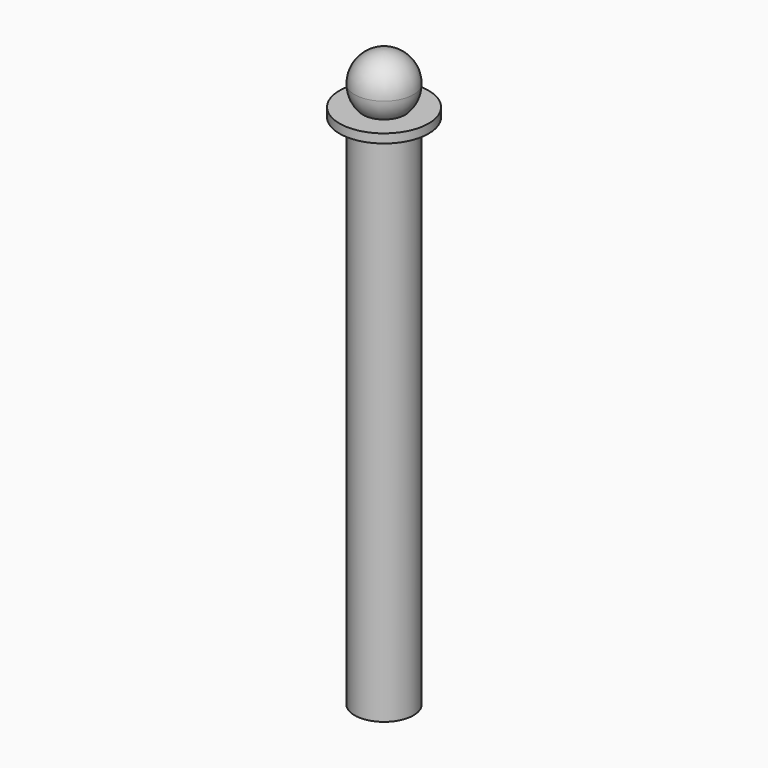
from build123d import *

# Parameters (mm, degrees)
F0_R     = 4.191
F1_DEPTH = 73.66
F2_R     = 4.191
F3_DEPTH = 8.382
F4_R     = 4.19099
F5_R     = 6.35
F6_DEPTH = 1.27
F7_R     = 1.905
F8_DEPTH = 12.7


# Not quite as in the source:
# - a fillet or chamfer is up to 0.001 mm smaller than in the source, because OpenCascade refuses the exact size


with BuildPart() as f1:
    # F0 (on Top) → F1 (new body)
    with BuildSketch(Plane.XY):
        Circle(F0_R)
    extrude(amount=F1_DEPTH)



with BuildPart() as f3:
    # F2 (on face) → F3 (new body)
    with BuildSketch(Plane.XY.offset(73.66)):
        Circle(F2_R)
    extrude(amount=F3_DEPTH)

    # F4 (radius 4.191 in the source; OpenCascade refuses exactly that, so slightly less here)
    f4_edges = [f3.edges().sort_by_distance(p)[0] for p in [
        (-4.191, 0, 73.66),
        (-4.191, 0, 82.042),
    ]]
    fillet(f4_edges, radius=F4_R)


with BuildPart() as f1_1:
    add(f1.part)

    add(f3.part)  # F6 merges F3
    # F5 (on face) → F6 (join)
    with BuildSketch(Plane.XY.offset(73.66)):
        Circle(F5_R)
    extrude(amount=F6_DEPTH)

    # F7 (on face) → F8 (cut)
    with BuildSketch(Plane(origin=(0, 0, 0), x_dir=(1, 0, 0), z_dir=(0, 0, -1))):
        Circle(F7_R)
    extrude(amount=-F8_DEPTH, mode=Mode.SUBTRACT)


solid = f1_1.part
